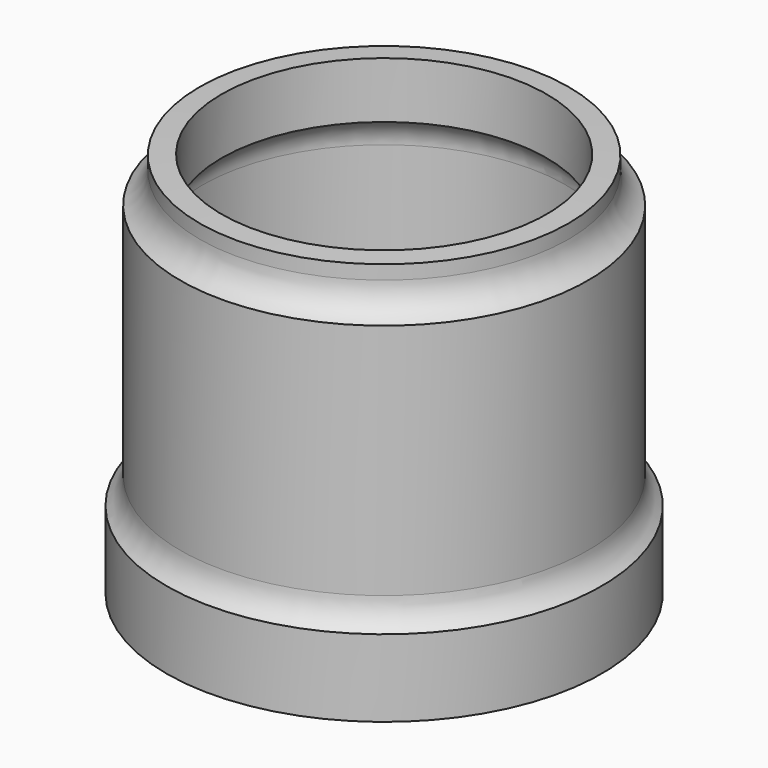
from build123d import *


# Not quite as in the source:
# - a fillet or chamfer that OpenCascade refuses, or shapes differently, is made with other operations: its cross-section is extruded or revolved along the edge and cut away or added


with BuildPart() as f1:
    # F0 (on Front) → F1 (revolve)
    with BuildSketch(Plane.XZ):
        Polygon((-16.5, 0), (-16.5, 5.7386059155), (-14.75, 5.7386059155), (-14.75, 10.8408229426), (-16.75, 10.7678563523), (-16.75, 6.7678563523), (-18.5, 6.7678563523), (-18.5, -17.2321436477), (-19.75, -17.2321436477), (-19.75, -24.2321436477), (-17.75, -24.2321436477), (-17.75, -17.2321436477), (-16.5, -17.2300804406), align=None)
    revolve(axis=Axis((0, 0, -1.1706372043), (0, 0, -1)))

    # F2: fillet of radius 3 on 4 edges, made by hand

    # F2_s1 → F2_t2 (revolve)
    with BuildSketch(Plane.XZ):
        with BuildLine():
            ThreePointArc((-18.5, 6.7678563523), (-17.2251237654, 7.8748492064), (-16.75, 9.495034381))
            Line((-16.75, 9.495034381), (-16.75, 6.7678563523))
            Line((-16.75, 6.7678563523), (-18.5, 6.7678563523))
        make_face()
    revolve(axis=Axis((0, 0, 6.7678563523), (0, 0, -1)))

    # F2_s3 → F2_t4 (revolve)
    with BuildSketch(Plane.XZ):
        with BuildLine():
            ThreePointArc((-19.75, -17.2321436477), (-18.830730437, -16.1647514552), (-18.5, -14.7954450615))
            Line((-18.5, -14.7954450615), (-18.5, -17.2321436477))
            Line((-18.5, -17.2321436477), (-19.75, -17.2321436477))
        make_face()
    revolve(axis=Axis((0, 0, -17.2321436477), (0, 0, -1)))

    # F2_s5 → F2_t6 (revolve)
    with BuildSketch(Plane.XZ):
        with BuildLine():
            ThreePointArc((-16.5, -17.2300804406), (-17.419269563, -18.2974726331), (-17.75, -19.6667790268))
            Line((-17.75, -19.6667790268), (-17.75, -17.2321436477))
            Line((-17.75, -17.2321436477), (-16.5, -17.2300804406))
        make_face()
    revolve(axis=Axis((0, 0, -17.2321436477), (0, 0, -1)))

    # F2_s7 → F2_t8 (revolve)
    with BuildSketch(Plane.XZ):
        with BuildLine():
            ThreePointArc((-16.5, 3.0114278869), (-16.0248762346, 4.6316130615), (-14.75, 5.7386059155))
            Line((-14.75, 5.7386059155), (-16.5, 5.7386059155))
            Line((-16.5, 5.7386059155), (-16.5, 3.0114278869))
        make_face()
    revolve(axis=Axis((0, 0, 5.7386059155), (0, 0, -1)))


solid = f1.part
